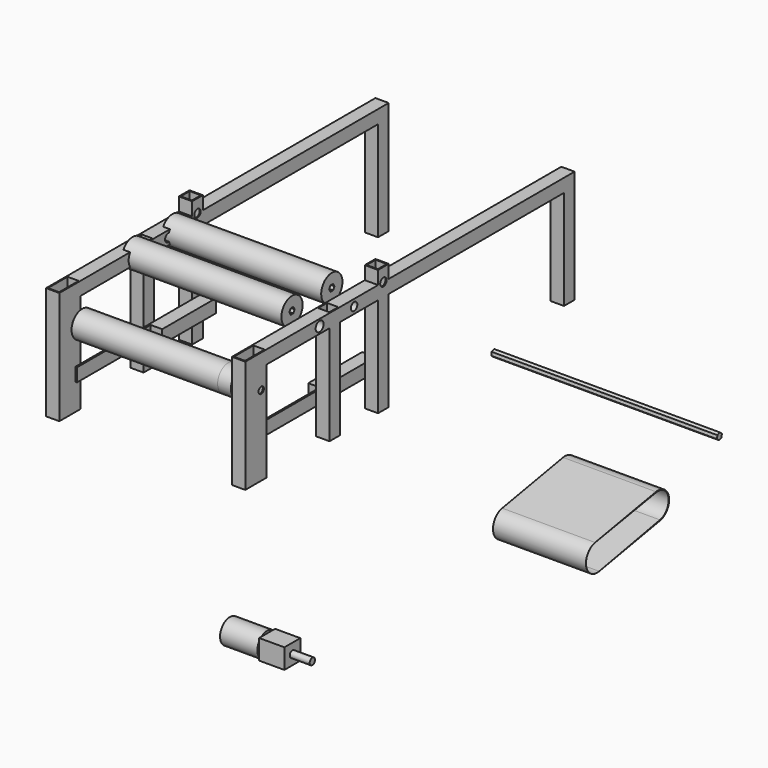
from build123d import *

# Parameters (mm, degrees)
F2_R      = 25.4
F3_DEPTH  = 304.8
F0_W      = 150.642607832
F0_H      = 25.4
F0_R      = 9.525
F0_W_2    = 25.4
F0_W_3    = 90.657392168
F0_R_2    = 7.62
F0_H_2    = 190.5
F0_R_3    = 6.35
F0_W_4    = 419.1
F4_DEPTH  = 25.4
F6_DEPTH  = 279.4
F7_DEPTH  = 25.4
F9_DEPTH  = 431.8
F10_W     = 90.657392168
F10_H     = 25.4
F10_W_2   = 25.4
F10_W_3   = 12.7
F11_DEPTH = 25.4
F12_W     = 150.642607832
F12_H     = 25.4
F12_W_2   = 12.7
F13_DEPTH = 3.175
F14_W     = 21.336
F14_H     = 21.336
F15_DEPTH = 241.3
F16_W     = 21.336
F16_H     = 21.336
F17_DEPTH = 215.9
F18_W     = 21.336
F18_H     = 46.736
F19_DEPTH = 215.9
F22_DEPTH = 177.8
F23_R     = 23.495
F24_DEPTH = 71.374
F25_R     = 2.5019
F26_DEPTH = 7.62
F27_R     = 2.5019
F28_DEPTH = 48.26
F29_R     = 6.35
F29_R_2   = 2.5019
F30_DEPTH = 38.1


# Not quite as in the source:
# - a length typed as a fraction of an inch, garbled in the dataset ("3 / 203.2 mm" for 3/8 in), is restored


with BuildPart() as f3:
    # F2 (on offset) → F3 (new body)
    with BuildSketch(Plane.YZ.offset(-63.5)):
        with Locations((-281.3588317816, 191.0254396081)):
            Circle(F2_R)
        Polygon((-275.0088317816, 191.0254396081), (-278.1838317816, 185.5261782941), (-284.5338317816, 185.5261782941), (-287.7088317816, 191.0254396081), (-284.5338317816, 196.5247009221), (-278.1838317816, 196.5247009221), align=None, mode=Mode.SUBTRACT)
    extrude(amount=-F3_DEPTH)


with BuildPart() as f3b:
    # F2 (on offset) → F3, piece 2 (new body)
    with BuildSketch(Plane.YZ.offset(-63.5)):
        with Locations((-186.1088317816, 191.0254396081)):
            Circle(F2_R)
        Polygon((-179.7588317816, 191.0254396081), (-182.9338317816, 185.5261782941), (-189.2838317816, 185.5261782941), (-192.4588317816, 191.0254396081), (-189.2838317816, 196.5247009221), (-182.9338317816, 196.5247009221), align=None, mode=Mode.SUBTRACT)
    extrude(amount=-F3_DEPTH)


with BuildPart() as f4:
    # F0 (on Right) → F4 (new body)
    with BuildSketch(Plane.YZ):
        with Locations((-346.3255038977, 191.0254396081)):
            Rectangle(F0_W, F0_H)
        with Locations((-294.6468078136, 191.0254396081)):
            Circle(F0_R, mode=Mode.SUBTRACT)
        with Locations((-258.3041999817, 191.0254396081)):
            Rectangle(F0_W_2, F0_H)
        with Locations((-200.2755038977, 191.0254396081)):
            Rectangle(F0_W_3, F0_H)
        with Locations((-212.0968078136, 191.0254396081)):
            Circle(F0_R_2, mode=Mode.SUBTRACT)
        with Locations((-142.2468078136, 83.0754396081)):
            Rectangle(F0_W_2, F0_H_2)
        Polygon((-472.4468078136, 203.7254396081), (-472.4468078136, -12.1745603919), (-421.6468078136, -12.1745603919), (-421.6468078136, 178.3254396081), (-421.6468078136, 203.7254396081), align=None)
        with Locations((-434.3468078136, 140.2254396081)):
            Circle(F0_R_3, mode=Mode.SUBTRACT)
        with BuildLine():
            Line((-154.9468078136, 229.1254396081), (-154.9468078136, 203.7254396081))
            Line((-154.9468078136, 203.7254396081), (-149.8668078136, 203.7254396081))
            ThreePointArc((-149.8668078136, 203.7254396081), (-142.2468078136, 211.3454396081), (-134.6268078136, 203.7254396081))
            Line((-134.6268078136, 203.7254396081), (-129.5468078136, 203.7254396081))
            Line((-129.5468078136, 203.7254396081), (-129.5468078136, 229.1254396081))
            Line((-129.5468078136, 229.1254396081), (-154.9468078136, 229.1254396081))
        make_face()
        with Locations((302.2531921864, 191.0254396081)):
            Rectangle(F0_W_2, F0_H)
        with Locations((-258.3041999817, 83.0754396081)):
            Rectangle(F0_W_2, F0_H_2)
        with BuildLine():
            Line((-149.8668078136, 203.7254396081), (-154.9468078136, 203.7254396081))
            Line((-154.9468078136, 203.7254396081), (-154.9468078136, 178.3254396081))
            Line((-154.9468078136, 178.3254396081), (-129.5468078136, 178.3254396081))
            Line((-129.5468078136, 178.3254396081), (-129.5468078136, 203.7254396081))
            Line((-129.5468078136, 203.7254396081), (-134.6268078136, 203.7254396081))
            ThreePointArc((-134.6268078136, 203.7254396081), (-142.2468078136, 196.1054396081), (-149.8668078136, 203.7254396081))
        make_face()
        with Locations((80.0031921864, 191.0254396081)):
            Rectangle(F0_W_4, F0_H)
        with Locations((302.2531921864, 83.0754396081)):
            Rectangle(F0_W_2, F0_H_2)
    extrude(amount=-F4_DEPTH)

    # F10 (on face) → F11 (join)
    with BuildSketch(Plane(origin=(-25.4, 0, 0), x_dir=(0, -1, 0), z_dir=(-1, 0, 0))):
        with Locations((200.2755038977, 51.3254396081)):
            Rectangle(F10_W, F10_H)
        with Locations((142.2468078136, 51.3254396081)):
            Rectangle(F10_W_2, F10_H)
        with Locations((251.9541999817, 51.3254396081)):
            Rectangle(F10_W_3, F10_H)
    extrude(amount=F11_DEPTH)

    # F12 (on face) → F13 (join)
    with BuildSketch(Plane(origin=(-25.4, 0, 0), x_dir=(0, -1, 0), z_dir=(-1, 0, 0))):
        with Locations((346.3255038977, 51.3254396081)):
            Rectangle(F12_W, F12_H)
        with Locations((427.9968078136, 51.3254396081)):
            Rectangle(F12_W_2, F12_H)
        with Locations((264.6541999817, 51.3254396081)):
            Rectangle(F12_W_2, F12_H)
    extrude(amount=F13_DEPTH)

    # F14 (on face) → F15 (cut, through all)
    with BuildSketch(Plane(origin=(0, 0, -12.1745603919), x_dir=(1, 0, 0), z_dir=(0, 0, -1))):
        with Locations((-12.7, 142.2468078136)):
            Rectangle(F14_W, F14_H)
    extrude(amount=-F15_DEPTH, mode=Mode.SUBTRACT)

    # F16 (on face) → F17 (cut, through all)
    with BuildSketch(Plane(origin=(0, 0, -12.1745603919), x_dir=(1, 0, 0), z_dir=(0, 0, -1))):
        with Locations((-12.7, 258.3041999817)):
            Rectangle(F16_W, F16_H)
    extrude(amount=-F17_DEPTH, mode=Mode.SUBTRACT)

    # F18 (on face) → F19 (cut, through all)
    with BuildSketch(Plane(origin=(0, 0, -12.1745603919), x_dir=(1, 0, 0), z_dir=(0, 0, -1))):
        with Locations((-12.7, 447.0468078136)):
            Rectangle(F18_W, F18_H)
    extrude(amount=-F19_DEPTH, mode=Mode.SUBTRACT)


with BuildPart() as f6:
    # F2 (on offset) → F6 (new body)
    with BuildSketch(Plane.YZ.offset(-63.5)):
        with Locations((-433.7588317816, 140.2254396081)):
            Circle(F2_R)
        Polygon((-427.4088317816, 140.2254396081), (-430.5838317816, 134.7261782941), (-436.9338317816, 134.7261782941), (-440.1088317816, 140.2254396081), (-436.9338317816, 145.7247009221), (-430.5838317816, 145.7247009221), align=None, mode=Mode.SUBTRACT)
    extrude(amount=-F6_DEPTH)

    # F2 (on offset) → F7 (join)
    with BuildSketch(Plane.YZ.offset(-63.5)):
        with Locations((-433.7588317816, 140.2254396081)):
            Circle(F2_R)
        Polygon((-427.4088317816, 140.2254396081), (-430.5838317816, 134.7261782941), (-436.9338317816, 134.7261782941), (-440.1088317816, 140.2254396081), (-436.9338317816, 145.7247009221), (-430.5838317816, 145.7247009221), align=None, mode=Mode.SUBTRACT)
    extrude(amount=F7_DEPTH)


with BuildPart() as f9:
    # F8 (on Right) → F9 (new body)
    with BuildSketch(Plane.YZ):
        Polygon((120.6004723048, -29.2308382335), (126.5187017848, -26.9293040012), (127.4846294119, -20.65319981), (122.532327559, -16.6786298511), (116.6140980791, -18.9801640834), (115.648170452, -25.2562682746), align=None)
    extrude(amount=F9_DEPTH)


with BuildPart() as f20_1:
    # F20: instance of F4
    add(f4.part.mirror(Plane.YZ.offset(-190.5)))


with BuildPart() as f22:
    # F21 (on Right) → F22 (new body)
    with BuildSketch(Plane.YZ):
        with BuildLine():
            ThreePointArc((141.8123362125, -292.6105024954), (120.2965632809, -323.5887095958), (151.2747703813, -345.1044825274))
            Line((151.2747703813, -345.1044825274), (296.8830721368, -318.8574925114))
            ThreePointArc((296.8830721368, -318.8574925114), (318.3988450683, -287.879285411), (287.4206379679, -266.3635124794))
            Line((287.4206379679, -266.3635124794), (141.8123362125, -292.6105024954))
        make_face()
        with BuildLine():
            ThreePointArc((287.8540655576, -267.5767451773), (317.1489884009, -288.1045814626), (296.8655957088, -317.5692814924))
            Line((296.8655957088, -317.5692814924), (151.4857400561, -345.025870467))
            ThreePointArc((151.4857400561, -345.025870467), (120.3349621896, -323.5817879041), (142.0374763015, -292.6105024954))
            Line((142.0374763015, -292.6105024954), (287.8540655576, -267.5767451773))
        make_face(mode=Mode.SUBTRACT)
    extrude(amount=F22_DEPTH)


with BuildPart() as f24:
    # F23 (on Right) → F24 (new body)
    with BuildSketch(Plane.YZ):
        with Locations((-509.2304348946, -234.628289938)):
            Circle(F23_R)
    extrude(amount=F24_DEPTH)

    # F25 (on face) → F26 (join)
    with BuildSketch(Plane.YZ.offset(71.374)):
        with Locations((-509.2304348946, -234.628289938)):
            Circle(F25_R)
    extrude(amount=F26_DEPTH)

    # F27 (on face) → F28 (join)
    with BuildSketch(Plane.YZ.offset(71.374)):
        with BuildLine():
            Line((-495.5315494147, -215.540189938), (-522.9293203744, -215.540189938))
            ThreePointArc((-522.9293203744, -215.540189938), (-525.9485013077, -218.1200713665), (-528.4900418615, -221.1715977561))
            Line((-528.4900418615, -221.1715977561), (-528.4900418615, -248.0849821198))
            ThreePointArc((-528.4900418615, -248.0849821198), (-525.9941742028, -251.0901266947), (-523.0348792293, -253.640189938))
            Line((-523.0348792293, -253.640189938), (-495.4259905599, -253.640189938))
            ThreePointArc((-495.4259905599, -253.640189938), (-492.7196132543, -251.3437855562), (-490.3900418615, -248.6659042424))
            Line((-490.3900418615, -248.6659042424), (-490.3900418615, -220.5906756335))
            ThreePointArc((-490.3900418615, -220.5906756335), (-492.7659879565, -217.8671142028), (-495.5315494147, -215.540189938))
        make_face()
        with Locations((-509.2304348946, -234.628289938)):
            Circle(F27_R, mode=Mode.SUBTRACT)
        with BuildLine():
            Line((-522.9293203744, -215.540189938), (-528.4900418615, -215.540189938))
            Line((-528.4900418615, -215.540189938), (-528.4900418615, -221.1715977561))
            ThreePointArc((-528.4900418615, -221.1715977561), (-525.9485013077, -218.1200713665), (-522.9293203744, -215.540189938))
        make_face()
        with BuildLine():
            ThreePointArc((-523.0348792293, -253.640189938), (-525.9941742028, -251.0901266947), (-528.4900418615, -248.0849821198))
            Line((-528.4900418615, -248.0849821198), (-528.4900418615, -253.640189938))
            Line((-528.4900418615, -253.640189938), (-523.0348792293, -253.640189938))
        make_face()
        with BuildLine():
            Line((-490.3900418615, -253.640189938), (-490.3900418615, -248.6659042424))
            ThreePointArc((-490.3900418615, -248.6659042424), (-492.7196132543, -251.3437855562), (-495.4259905599, -253.640189938))
            Line((-495.4259905599, -253.640189938), (-490.3900418615, -253.640189938))
        make_face()
        with BuildLine():
            Line((-490.3900418615, -215.540189938), (-495.5315494147, -215.540189938))
            ThreePointArc((-495.5315494147, -215.540189938), (-492.7659879565, -217.8671142028), (-490.3900418615, -220.5906756335))
            Line((-490.3900418615, -220.5906756335), (-490.3900418615, -215.540189938))
        make_face()
    extrude(amount=F28_DEPTH)

    # F29 (on face) → F30 (join)
    with BuildSketch(Plane.YZ.offset(119.634)):
        with Locations((-509.2304348946, -234.628289938)):
            Circle(F29_R)
        with Locations((-509.2304348946, -234.628289938)):
            Circle(F29_R_2, mode=Mode.SUBTRACT)
        with Locations((-509.2304348946, -234.628289938)):
            Circle(F29_R_2)
    extrude(amount=F30_DEPTH)


solid = Compound([f3.part, f3b.part, f4.part, f6.part, f9.part, f20_1.part, f22.part, f24.part])
